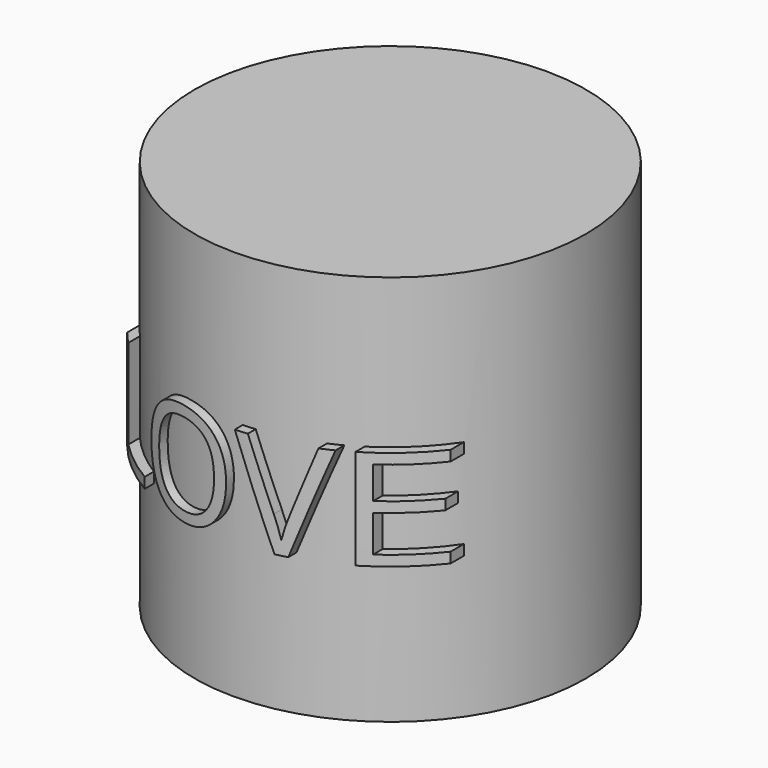
from build123d import *

# Parameters (mm, degrees)
F0_R         = 50
F1_DEPTH     = 100
F3_TEXT_SIZE = 35.8264686333
F4_DEPTH     = 46
F5_R         = 85.8106021113
F5_R_2       = 52.5
F6_DEPTH     = 104.3


# Not quite as in the source:
# - Text() gives the source's letters only with a copy of the font that has no kerning and outlines rounded to 1/6400 em; it was checked with that copy


with BuildPart() as f1:
    # F0 (on Top) → F1 (new body)
    with BuildSketch(Plane.XY):
        Circle(F0_R)
    extrude(amount=F1_DEPTH)

    # F3 (on offset) → F4 (join)
    with BuildSketch(Plane.XZ.offset(70)):
        with Locations((-44.2655980587, 36.2250842154)):
            Text('LOVE', F3_TEXT_SIZE, font='Open Sans', text_align=(TextAlign.LEFT, TextAlign.BOTTOM))
    extrude(amount=-F4_DEPTH)

    # F5 (on face) → F6 (cut)
    with BuildSketch(Plane.XY.offset(100)):
        Circle(F5_R)
        Circle(F5_R_2, mode=Mode.SUBTRACT)
    extrude(amount=-F6_DEPTH, mode=Mode.SUBTRACT)


solid = f1.part
